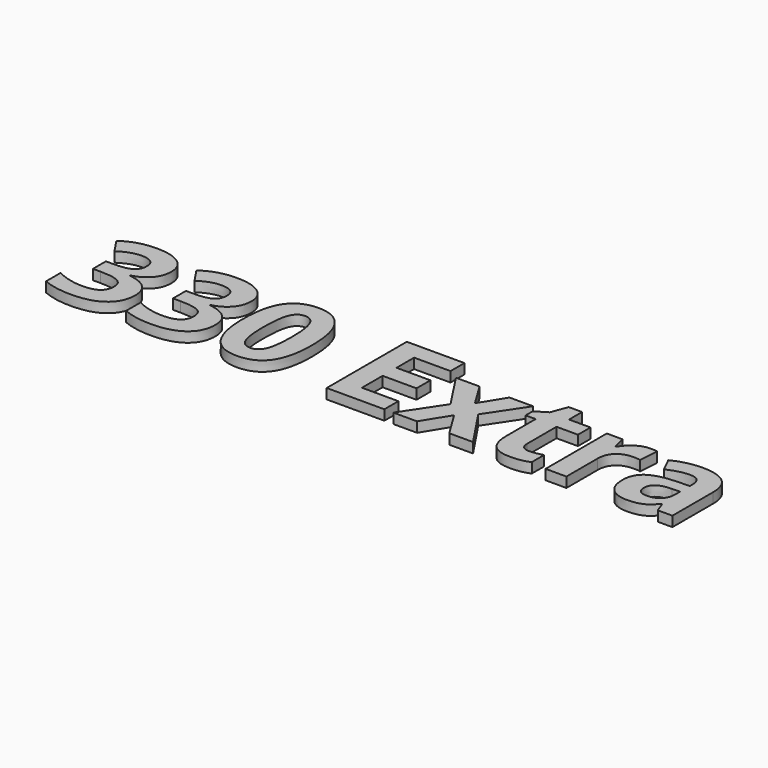
from build123d import *

# Parameters (mm, degrees)
F1_DEPTH     = 1.905
F2_R         = 1.27
F3_TEXT_SIZE = 17.6388888889
F4_DEPTH     = 1.27


# Not quite as in the source:
# - Text() gives the source's letters only with a copy of the font that has no kerning and outlines rounded to 1/6400 em; it was checked with that copy


with BuildPart() as f1:
    # F0 (on Top) → F1 (new body)
    with BuildSketch(Plane.XY):
        with BuildLine():
            add(Edge.make_bspline(
                [(-50.8, 0), (-44.583607465, 28.7666022778), (-33.2989580929, 72.5001161814), (0, 76.2)],
                knots=[0, 0, 0, 0, 91.5810023968, 91.5810023968, 91.5810023968, 91.5810023968], degree=3))
            Line((-50.8, 0), (-44.3035974861, 0))
            add(Edge.make_bspline(
                [(-44.3035974861, 0), (-44.1435779548, 0.7410345001), (-43.4394104299, 4.0010733535), (-41.8479460678, 11.2821500743), (-39.0720854967, 21.8066534177), (-35.2093555317, 33.5744319572), (-30.7181563408, 44.1297128959), (-25.7625794511, 52.439792295), (-21.1567773404, 58.0769214208), (-17.1166725863, 62.1241646605), (-13.1858587871, 65.1319016492), (-8.9410530969, 67.4891815532), (-4.8649357319, 69.0398398434), (-1.8187937025, 69.6063857314), (-0.3499831481, 69.7844553695), (0, 69.8215681813)],
                knots=[1.3722368836, 1.3722368836, 1.3722368836, 1.3722368836, 3.6465959369, 11.3775101917, 23.7303497403, 36.2811365397, 48.5097566878, 58.0688014534, 65.1942849024, 70.2950508117, 75.1952512239, 79.987609508, 84.8207106101, 88.200815676, 89.2566550269, 89.2566550269, 89.2566550269, 89.2566550269], degree=3))
            add(Edge.make_bspline(
                [(44.3035974861, 0), (44.1435779548, 0.7410345001), (43.4394104299, 4.0010733535), (41.8479460678, 11.2821500743), (39.0720854967, 21.8066534177), (35.2093555317, 33.5744319572), (30.7181563408, 44.1297128959), (25.7625794511, 52.439792295), (21.1567773404, 58.0769214208), (17.1166725863, 62.1241646605), (13.1858587871, 65.1319016492), (8.9410530969, 67.4891815532), (4.8649357319, 69.0398398434), (1.8187937025, 69.6063857314), (0.3499831481, 69.7844553695), (0, 69.8215681813)],
                knots=[1.3722368836, 1.3722368836, 1.3722368836, 1.3722368836, 3.6465959369, 11.3775101917, 23.7303497403, 36.2811365397, 48.5097566878, 58.0688014534, 65.1942849024, 70.2950508117, 75.1952512239, 79.987609508, 84.8207106101, 88.200815676, 89.2566550269, 89.2566550269, 89.2566550269, 89.2566550269], degree=3))
            Line((44.3035974861, 0), (50.8, 0))
            add(Edge.make_bspline(
                [(50.8, 0), (44.583607465, 28.7666022778), (33.2989580929, 72.5001161814), (0, 76.2)],
                knots=[0, 0, 0, 0, 91.5810023968, 91.5810023968, 91.5810023968, 91.5810023968], degree=3))
        make_face()
    extrude(amount=F1_DEPTH)

    # F2
    f2_edges = [f1.edges().sort_by_distance(p)[0] for p in [
        (-47.551799, 0, 1.905),
        (-36.081129, 46.470583, 1.905),
        (36.081129, 46.470583, 1.905),
        (47.551799, 0, 1.905),
        (31.502344, 41.95843, 1.905),
        (-31.502344, 41.95843, 1.905),
    ]]
    fillet(f2_edges, radius=F2_R)


with BuildPart() as f4:
    # F3 (on face) → F4 (new body)
    with BuildSketch(Plane.XY.offset(1.905)):
        with Locations((-40.4991644965, 7.62)):
            Text('330 Extra', F3_TEXT_SIZE, font='Open Sans', font_style=FontStyle.BOLD, text_align=(TextAlign.LEFT, TextAlign.BOTTOM))
    extrude(amount=F4_DEPTH)


solid = f4.part
